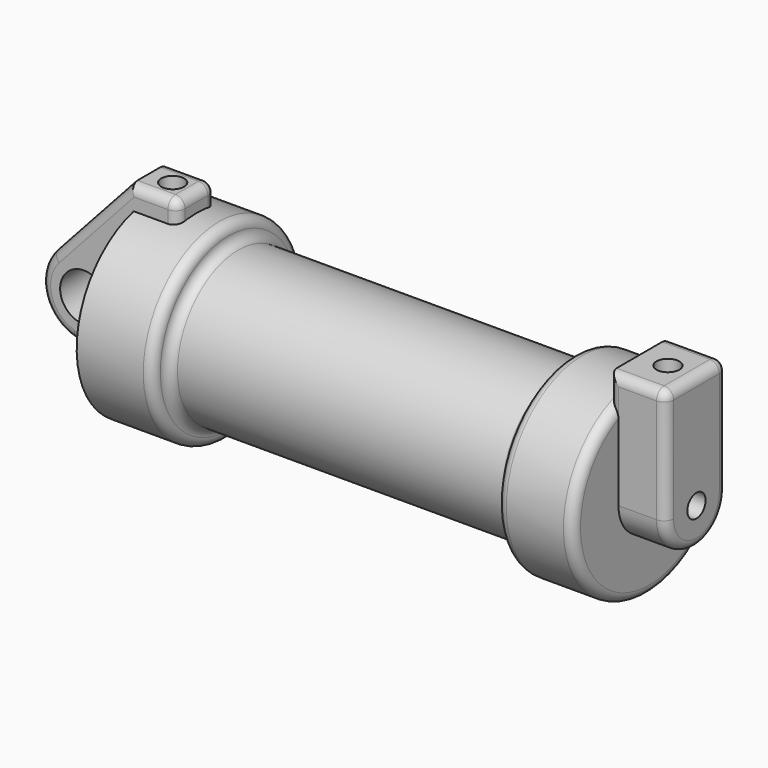
from build123d import *

# Parameters (mm, degrees)
F0_W      = 5.842
F0_H      = 12.7
F0_R      = 3.175
F2_DEPTH  = 3.175
F3_R      = 1.524
F4_DEPTH  = 1.27
F5_DEPTH  = 6.35
F6_DEPTH  = 56.134
F7_R      = 1.524
F8_DEPTH  = 17.78
F9_R      = 1.524
F10_DEPTH = 10.414
F11_R     = 1.26999
F11_2_R   = 1.26999
F11_3_R   = 1.26999


# Not quite as in the source:
# - a fillet or chamfer is up to 0.001 mm smaller than in the source, because OpenCascade refuses the exact size


with BuildPart() as f1:
    # F0 (on Front) → F1 (revolve)
    with BuildSketch(Plane.XZ):
        Polygon((5.842, 12.7), (5.842, 0), (66.294, 0), (66.294, 12.7), (56.134, 12.7), (56.134, 10.16), (10.16, 10.16), (10.16, 12.7), align=None)
        with Locations((2.921, 6.35)):
            Rectangle(F0_W, F0_H)
    revolve(axis=Axis((33.147, 0, 0), (-1, 0, 0)))

    # F3 (on face) → F6 (cut, through all)
    with BuildSketch(Plane.YZ.offset(66.294)):
        Circle(F3_R)
    extrude(amount=-F6_DEPTH, mode=Mode.SUBTRACT)

    # F11 (radius 1.27 in the source; OpenCascade refuses exactly that, so slightly less here)
    f11_edges = [f1.edges().sort_by_distance(p)[0] for p in [
        (10.16, 0, -12.7),
        (10.16, 0, -10.16),
        (56.134, 0, -12.7),
        (66.294, 0, -12.7),
        (66.294, -1.524, 0),
        (56.134, 0, -10.16),
    ]]
    fillet(f11_edges, radius=F11_R)


with BuildPart() as f2:
    # F0 (on Front) → F2 (new body, symmetric)
    with BuildSketch(Plane.XZ):
        with BuildLine():
            Line((-0.9398, 0), (0, 0))
            Line((0, 0), (0, 12.7))
            Line((0, 12.7), (5.842, 12.7))
            Line((5.842, 12.7), (5.842, 15.24))
            Line((5.842, 15.24), (-0.508, 15.24))
            Line((-0.508, 15.24), (-10.8806298187, 3.8475430269))
            ThreePointArc((-10.8806298187, 3.8475430269), (-4.5919612295, 5.3297205562), (-0.9398, 0))
        make_face()
        with BuildLine():
            ThreePointArc((-8.1826630726, -5.5069827884), (-3.1957909266, -4.5493385486), (-0.9398, 0))
            ThreePointArc((-0.9398, 0), (-4.5919612295, 5.3297205562), (-10.8806298187, 3.8475430269))
            ThreePointArc((-10.8806298187, 3.8475430269), (-12.1459778134, -1.5837270034), (-8.1826630726, -5.5069827884))
        make_face()
        with Locations((-6.6548, 0)):
            Circle(F0_R, mode=Mode.SUBTRACT)
        with BuildLine():
            Line((5.842, 0), (0, 0))
            Line((0, 0), (-0.9398, 0))
            ThreePointArc((-0.9398, 0), (-3.1957909266, -4.5493385486), (-8.1826630726, -5.5069827884))
            Line((-8.1826630726, -5.5069827884), (5.842, -9.398))
            Line((5.842, -9.398), (5.842, 0))
        make_face()
        with Locations((2.921, 6.35)):
            Rectangle(F0_W, F0_H)
    extrude(amount=F2_DEPTH, both=True)

    # F7 (on face) → F8 (cut)
    with BuildSketch(Plane.XY.offset(15.24)):
        with Locations((2.667, 0)):
            Circle(F7_R)
    extrude(amount=-F8_DEPTH, mode=Mode.SUBTRACT)

    # F11#2 (radius 1.27 in the source; OpenCascade refuses exactly that, so slightly less here)
    f11_2_edges = [f2.edges().sort_by_distance(p)[0] for p in [
        (5.842, 0, 15.24),
        (2.667, -3.175, 15.24),
        (2.667, 3.175, 15.24),
        (-5.694315, -3.175, 9.543772),
        (-12.145978, -3.175, -1.583727),
        (-5.694315, 3.175, 9.543772),
        (5.842, 3.175, 2.921),
        (5.842, -3.175, 2.921),
        (-12.145978, 3.175, -1.583727),
        (-1.170332, 3.175, -7.452491),
        (-1.170332, -3.175, -7.452491),
    ]]
    fillet(f11_2_edges, radius=F11_2_R)


with BuildPart() as f4:
    # F3 (on face) → F4 (new body)
    with BuildSketch(Plane.YZ.offset(66.294)):
        with BuildLine():
            ThreePointArc((-5.08, 11.6397422652), (0, 12.7), (5.08, 11.6397422652))
            Line((5.08, 11.6397422652), (5.08, 15.24))
            Line((5.08, 15.24), (-5.08, 15.24))
            Line((-5.08, 15.24), (-5.08, 11.6397422652))
        make_face()
        with BuildLine():
            ThreePointArc((-5.08, 0), (0, 5.08), (5.08, 0))
            Line((5.08, 0), (5.08, 11.6397422652))
            ThreePointArc((5.08, 11.6397422652), (0, 12.7), (-5.08, 11.6397422652))
            Line((-5.08, 11.6397422652), (-5.08, 0))
        make_face()
        with BuildLine():
            ThreePointArc((-5.08, 0), (0, -5.08), (5.08, 0))
            ThreePointArc((5.08, 0), (0, 5.08), (-5.08, 0))
        make_face()
        Circle(F3_R, mode=Mode.SUBTRACT)
    extrude(amount=-F4_DEPTH)

    # F5 (add): a face of the model
    f5_faces = [f4.faces().sort_by_distance(p)[0] for p in [
        (66.294, 0, 5.8085929676),
    ]]
    extrude(f5_faces, amount=F5_DEPTH)

    # F9 (on face) → F10 (cut)
    with BuildSketch(Plane.XY.offset(15.24)):
        with Locations((68.834, 0)):
            Circle(F9_R)
    extrude(amount=-F10_DEPTH, mode=Mode.SUBTRACT)

    # F11#3 (radius 1.27 in the source; OpenCascade refuses exactly that, so slightly less here)
    f11_3_edges = [f4.edges().sort_by_distance(p)[0] for p in [
        (72.644, 0, 15.24),
        (68.834, 5.08, 15.24),
        (68.834, -5.08, 15.24),
        (72.644, -5.08, 7.62),
        (68.834, -5.08, 0),
        (65.024, 0, -5.08),
        (68.834, 5.08, 0),
        (72.644, 0, -5.08),
        (65.024, -5.08, 7.62),
        (65.024, 5.08, 7.62),
        (72.644, 5.08, 7.62),
    ]]
    fillet(f11_3_edges, radius=F11_3_R)


solid = Compound([f1.part, f2.part, f4.part])
